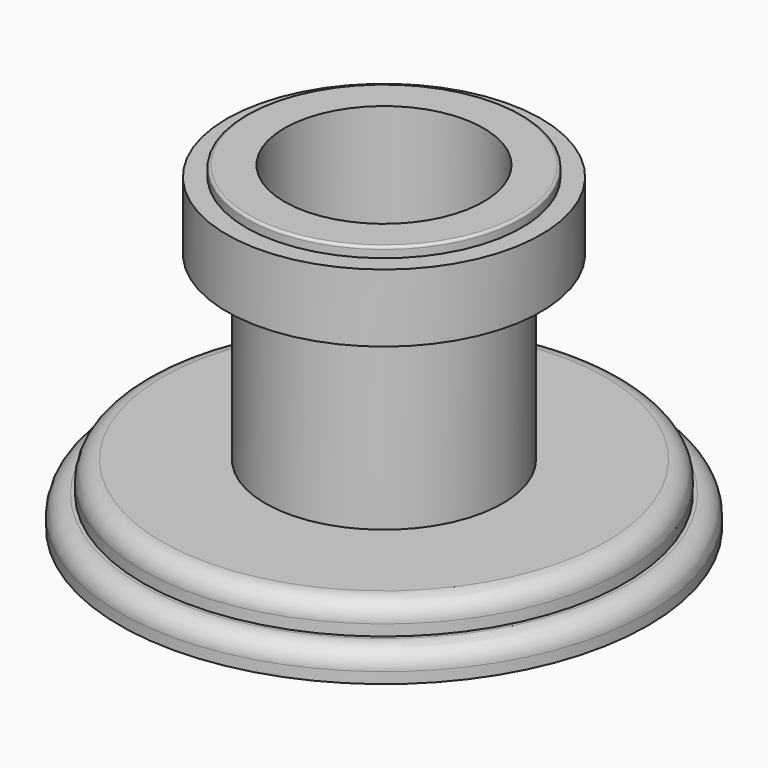
from build123d import *

# Parameters (mm, degrees)
F2_R = 1.27
F3_R = 0.50799


# Not quite as in the source:
# - a fillet or chamfer is up to 0.001 mm smaller than in the source, because OpenCascade refuses the exact size


with BuildPart() as f1:
    # F0 (on Front) → F1 (revolve)
    with BuildSketch(Plane.XZ):
        with BuildLine():
            Line((-17.5, 0), (-6.604, 0))
            Line((-6.604, 0), (-6.604, 21.1916357695))
            Line((-6.604, 21.1916357695), (-8.9683642305, 21.1916357695))
            ThreePointArc((-8.9683642305, 21.1916357695), (-9.0925574741, 21.1401932437), (-9.144, 21.016))
            Line((-9.144, 21.016), (-9.144, 20.508))
            Line((-9.144, 20.508), (-10.414, 20.508))
            Line((-10.414, 20.508), (-10.414, 16.008))
            Line((-10.414, 16.008), (-9.144, 16.008))
            Line((-9.144, 16.008), (-9.144, 15.5))
            Line((-9.144, 15.5), (-7.874, 15.5))
            Line((-7.874, 15.5), (-7.874, 4))
            Line((-7.874, 4), (-16, 4))
            Line((-16, 4), (-16, 2))
            Line((-16, 2), (-17.5, 2))
            Line((-17.5, 2), (-17.5, 0))
        make_face()
    revolve(axis=Axis((0, 0, 10.5958178848), (0, 0, -1)))

    # F2
    f2_edges = [f1.edges().sort_by_distance(p)[0] for p in [
        (16, 0, 4),
        (17.5, 0, 2),
    ]]
    fillet(f2_edges, radius=F2_R)

    # F3 (radius 0.508 in the source; OpenCascade refuses exactly that, so slightly less here)
    f3_edges = [f1.edges().sort_by_distance(p)[0] for p in [
        (9.144, 0, 15.5),
    ]]
    fillet(f3_edges, radius=F3_R)


solid = f1.part
